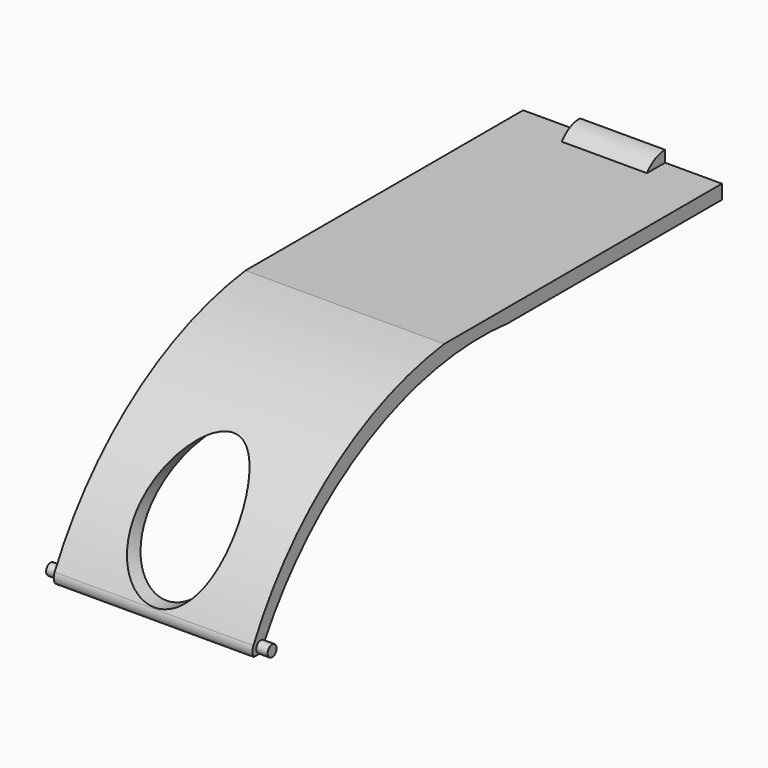
from build123d import *

# Parameters (mm, degrees)
F0_W          = 35
F0_H          = 57
F1_DEPTH      = 31.5
F4_DEPTH      = 57.001
F5_DEPTH      = 35.0010001
F7_DEPTH      = 35.0010001
F9_DEPTH      = 2
F9_DEPTH_BACK = 37
F11_DEPTH     = 37.001
F12_DEPTH     = 47
F13_W         = 15
F13_H         = 4
F14_DEPTH     = 2
F15_T1_DEPTH  = 35
F16_W         = 11
F16_H         = 1
F17_DEPTH     = 1


# Not quite as in the source:
# - a fillet or chamfer that OpenCascade refuses, or shapes differently, is made with other operations: its cross-section is extruded or revolved along the edge and cut away or added


with BuildPart() as f1:
    # F0 (on Top) → F1 (new body)
    with BuildSketch(Plane.XY):
        with Locations((0.0945744105, -24.8016776452)):
            Rectangle(F0_W, F0_H)
    extrude(amount=F1_DEPTH)

    # F3 (on face) → F4 (cut, through all)
    with BuildSketch(Plane.XZ.offset(53.3016776452)):
        with BuildLine():
            add(Edge.make_bspline(
                [(0.0945744105, 2), (14.3839935729, 2), (7.2392839917, 17), (0.0945744105, 32), (-7.0501351708, 17), (-14.194844752, 2), (0.0945744105, 2)],
                knots=[0, 0, 0, 2.0943951024, 2.0943951024, 4.1887902048, 4.1887902048, 6.2831853072, 6.2831853072, 6.2831853072], degree=2, weights=[1, 0.5, 1, 0.5, 1, 0.5, 1]))
        make_face()
    extrude(amount=-F4_DEPTH, mode=Mode.SUBTRACT)

    # F2 (on face) → F5 (cut, through all)
    with BuildSketch(Plane.YZ.offset(17.5945744105)):
        with BuildLine():
            ThreePointArc((-53.3016776452, 0), (-35.9248296563, 21.279893434), (-10.4231016291, 31.5))
            Line((-10.4231016291, 31.5), (-53.3016776452, 31.5))
            Line((-53.3016776452, 31.5), (-53.3016776452, 0))
        make_face()
    extrude(amount=-F5_DEPTH, mode=Mode.SUBTRACT)

    # F6 (on face) → F7 (cut, through all)
    with BuildSketch(Plane.YZ.offset(17.5945744105)):
        with BuildLine():
            Line((3.6983223548, 0), (3.6983223548, 29))
            ThreePointArc((3.6983223548, 29), (-28.0042777095, 22.8678173622), (-50.8016776452, 0))
            Line((-50.8016776452, 0), (3.6983223548, 0))
        make_face()
    extrude(amount=-F7_DEPTH, mode=Mode.SUBTRACT)

    # F8 (on face) → F9 (join, two sides)
    with BuildSketch(Plane.YZ.offset(17.5945744105)) as f9_sk:
        with BuildLine():
            ThreePointArc((-49.9582016017, 1.5371667936), (-51.6783665277, 1.4810577961), (-50.8016776452, 0))
            ThreePointArc((-50.8016776452, 0), (-50.3860655446, 0.7719448198), (-49.9582016017, 1.5371667936))
        make_face()
        with BuildLine():
            ThreePointArc((-49.9582016017, 1.5371667936), (-50.3860655446, 0.7719448198), (-50.8016776452, 0))
            ThreePointArc((-50.8016776452, 0), (-50.094570864, 0.2928932188), (-49.8016776452, 1))
            ThreePointArc((-49.8016776452, 1), (-49.8416057615, 1.2797534241), (-49.9582016017, 1.5371667936))
        make_face()
    extrude(amount=F9_DEPTH)
    extrude(f9_sk.sketch, amount=-F9_DEPTH_BACK)

    # F10 (on face) → F11 (cut, through all)
    with BuildSketch(Plane.YZ.offset(17.5945744105)):
        with BuildLine():
            Line((-53.3016776452, 0), (-52.3163572735, 0))
            ThreePointArc((-52.3163572735, 0), (-52.6137174082, 0.8962393447), (-52.4206060402, 1.8205639696))
            ThreePointArc((-52.4206060402, 1.8205639696), (-52.8695111773, 0.9143323688), (-53.3016776452, 0))
        make_face()
    extrude(amount=-F11_DEPTH, mode=Mode.SUBTRACT)

    # F12 (add): a face of the model
    f12_faces = [f1.faces().sort_by_distance(p)[0] for p in [
        (0.0945744105, 3.6983223548, 30.25),
    ]]
    extrude(f12_faces, amount=F12_DEPTH)

    # F13 (on face) → F14 (join)
    with BuildSketch(Plane.XY.offset(31.5)):
        with Locations((0.0945744105, 48.6983223548)):
            Rectangle(F13_W, F13_H)
    extrude(amount=F14_DEPTH)

    # F15: fillet of radius 5 on 1 edges, made by hand

    # F15_s2 → F15_t1 (cut)
    with BuildSketch(Plane.YZ.offset(-17.4054255895)):
        with BuildLine():
            ThreePointArc((46.6983223548, 31.5), (48.4622543773, 32.972135955), (50.6983223548, 33.5))
            Line((50.6983223548, 33.5), (46.6983223548, 33.5))
            Line((46.6983223548, 33.5), (46.6983223548, 31.5))
        make_face()
    extrude(amount=F15_T1_DEPTH, mode=Mode.SUBTRACT)

    # F16 (on face) → F17 (cut)
    with BuildSketch(Plane(origin=(0, 50.6983223548, 0), x_dir=(-1, 0, 0), z_dir=(0, 1, 0))):
        with Locations((-0.0945744105, 32.5)):
            Rectangle(F16_W, F16_H)
    extrude(amount=-F17_DEPTH, mode=Mode.SUBTRACT)


solid = f1.part
